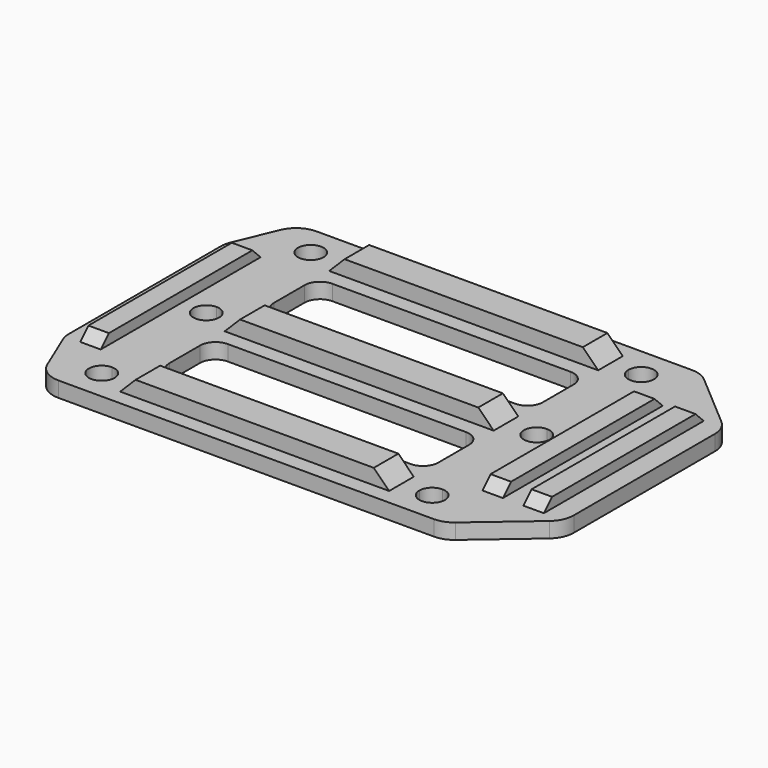
from build123d import *

# Parameters (mm, degrees)
F0_W       = 52.5
F0_H       = 3
F1_DEPTH   = 6
F0_H_2     = 6
F2_DEPTH   = 3
F4_SIZE    = 2.99999
F5_SIZE2   = 6
F5_SIZE    = 12
F5_2_SIZE2 = 6
F5_2_SIZE  = 12
F6_W       = 4
F6_H       = 39
F7_DEPTH   = 2
F8_SIZE    = 1.99999
F10_DEPTH  = 3
F13_DEPTH  = 3
F12_W      = 4
F12_H      = 39
F15_DEPTH  = 2
F16_SIZE   = 1.99999
F17_SIZE   = 1.99999
F18_DEPTH  = 25
F19_R      = 5


# Not quite as in the source:
# - a fillet or chamfer is up to 0.001 mm smaller than in the source, because OpenCascade refuses the exact size


with BuildPart() as f1:
    # F0 (on Top) → F1 (new body)
    with BuildSketch(Plane.XY):
        with Locations((0, 27)):
            Rectangle(F0_W, F0_H)
        with Locations((0, 24)):
            Rectangle(F0_W, F0_H)
    extrude(amount=F1_DEPTH)


with BuildPart() as f1b:
    # F0 (on Top) → F1, piece 2 (new body)
    with BuildSketch(Plane.XY):
        Rectangle(F0_W, F0_H_2)
    extrude(amount=F1_DEPTH)


with BuildPart() as f1c:
    # F0 (on Top) → F1, piece 3 (new body)
    with BuildSketch(Plane.XY):
        with Locations((0, -24)):
            Rectangle(F0_W, F0_H)
        with Locations((0, -27)):
            Rectangle(F0_W, F0_H)
    extrude(amount=F1_DEPTH)


with BuildPart() as f2:
    # F0 (on Top) → F2 (new body)
    with BuildSketch(Plane.XY):
        Polygon((-38.25, 28.5), (-38.25, -28.5), (-38.25, -31.5), (-35.25, -31.5), (35.25, -31.5), (38.25, -31.5), (38.25, -28.5), (38.25, 28.5), (38.25, 31.5), (35.25, 31.5), (-35.25, 31.5), (-38.25, 31.5), align=None)
        with BuildLine():
            Line((-26.25, -25.5), (-29.75, -25.5))
            ThreePointArc((-29.75, -25.5), (-34.017766953, -27.267766953), (-32.25, -23))
            Line((-32.25, -23), (-32.25, -2.5))
            ThreePointArc((-32.25, -2.5), (-34.75, 0), (-32.25, 2.5))
            Line((-32.25, 2.5), (-32.25, 23))
            ThreePointArc((-32.25, 23), (-34.017766953, 27.267766953), (-29.75, 25.5))
            Line((-29.75, 25.5), (-26.25, 25.5))
            Line((-26.25, 25.5), (-26.25, 28.5))
            Line((-26.25, 28.5), (26.25, 28.5))
            Line((26.25, 28.5), (26.25, 25.5))
            Line((26.25, 25.5), (29.75, 25.5))
            ThreePointArc((29.75, 25.5), (32.25, 28), (34.75, 25.5))
            ThreePointArc((34.75, 25.5), (34.017766953, 23.732233047), (32.25, 23))
            Line((32.25, 23), (32.25, 2.5))
            ThreePointArc((32.25, 2.5), (34.017766953, 1.767766953), (34.75, 0))
            ThreePointArc((34.75, 0), (34.017766953, -1.767766953), (32.25, -2.5))
            Line((32.25, -2.5), (32.25, -23))
            ThreePointArc((32.25, -23), (34.017766953, -23.732233047), (34.75, -25.5))
            ThreePointArc((34.75, -25.5), (32.25, -28), (29.75, -25.5))
            Line((29.75, -25.5), (26.25, -25.5))
            Line((26.25, -25.5), (26.25, -28.5))
            Line((26.25, -28.5), (-26.25, -28.5))
            Line((-26.25, -28.5), (-26.25, -25.5))
        make_face(mode=Mode.SUBTRACT)
        with BuildLine():
            ThreePointArc((-32.25, -23), (-30.482233047, -23.732233047), (-29.75, -25.5))
            Line((-29.75, -25.5), (-26.25, -25.5))
            Line((-26.25, -25.5), (-26.25, -22.5))
            Line((-26.25, -22.5), (26.25, -22.5))
            Line((26.25, -22.5), (26.25, -25.5))
            Line((26.25, -25.5), (29.75, -25.5))
            ThreePointArc((29.75, -25.5), (30.482233047, -23.732233047), (32.25, -23))
            Line((32.25, -23), (32.25, -2.5))
            ThreePointArc((32.25, -2.5), (29.75, 0), (32.25, 2.5))
            Line((32.25, 2.5), (32.25, 23))
            ThreePointArc((32.25, 23), (30.482233047, 23.732233047), (29.75, 25.5))
            Line((29.75, 25.5), (26.25, 25.5))
            Line((26.25, 25.5), (26.25, 22.5))
            Line((26.25, 22.5), (-26.25, 22.5))
            Line((-26.25, 22.5), (-26.25, 25.5))
            Line((-26.25, 25.5), (-29.75, 25.5))
            ThreePointArc((-29.75, 25.5), (-30.482233047, 23.732233047), (-32.25, 23))
            Line((-32.25, 23), (-32.25, 2.5))
            ThreePointArc((-32.25, 2.5), (-30.482233047, 1.767766953), (-29.75, 0))
            ThreePointArc((-29.75, 0), (-30.482233047, -1.767766953), (-32.25, -2.5))
            Line((-32.25, -2.5), (-32.25, -23))
        make_face()
        with BuildLine():
            ThreePointArc((-23.25, -19.5), (-25.3713203436, -18.6213203436), (-26.25, -16.5))
            Line((-26.25, -16.5), (-26.25, -9))
            ThreePointArc((-26.25, -9), (-25.3713203436, -6.8786796564), (-23.25, -6))
            Line((-23.25, -6), (23.25, -6))
            ThreePointArc((23.25, -6), (25.3713203436, -6.8786796564), (26.25, -9))
            Line((26.25, -9), (26.25, -16.5))
            ThreePointArc((26.25, -16.5), (25.3713203436, -18.6213203436), (23.25, -19.5))
            Line((23.25, -19.5), (-23.25, -19.5))
        make_face(mode=Mode.SUBTRACT)
        Rectangle(F0_W, F0_H_2, mode=Mode.SUBTRACT)
        with BuildLine():
            Line((-23.25, 19.5), (23.25, 19.5))
            ThreePointArc((23.25, 19.5), (25.3713203436, 18.6213203436), (26.25, 16.5))
            Line((26.25, 16.5), (26.25, 9))
            ThreePointArc((26.25, 9), (25.3713203436, 6.8786796564), (23.25, 6))
            Line((23.25, 6), (-23.25, 6))
            ThreePointArc((-23.25, 6), (-25.3713203436, 6.8786796564), (-26.25, 9))
            Line((-26.25, 9), (-26.25, 16.5))
            ThreePointArc((-26.25, 16.5), (-25.3713203436, 18.6213203436), (-23.25, 19.5))
        make_face(mode=Mode.SUBTRACT)
        Polygon((-38.25, -31.5), (-38.25, -28.5), (-38.25, 28.5), (-38.25, 31.5), (-41.25, 31.5), (-44.25, 31.5), (-44.25, 28.5), (-44.25, -28.5), (-44.25, -31.5), (-41.25, -31.5), align=None)
        Polygon((38.25, -28.5), (38.25, -31.5), (41.25, -31.5), (44.25, -31.5), (44.25, -28.5), (44.25, 28.5), (44.25, 31.5), (41.25, 31.5), (38.25, 31.5), (38.25, 28.5), align=None)
    extrude(amount=F2_DEPTH)


with BuildPart() as f1c_1:
    add(f1c.part)

    # F3: union F1, F1b, F2
    add(f1.part)
    add(f1b.part)
    add(f2.part)

    # F4 (size 3 in the source; OpenCascade refuses exactly that, so slightly less here)
    f4_edges = [f1c_1.edges().sort_by_distance(p)[0] for p in [
        (26.25, 25.5, 6),
        (26.25, 0, 6),
        (26.25, -25.5, 6),
        (-26.25, 25.5, 6),
        (-26.25, 0, 6),
        (-26.25, -25.5, 6),
    ]]
    chamfer(f4_edges, length=F4_SIZE)

    # F5
    f5_edges = [f1c_1.edges().sort_by_distance(p)[0] for p in [
        (44.25, -31.5, 1.5),
        (44.25, 31.5, 1.5),
    ]]
    f5_side = f1c_1.faces().sort_by_distance((44.25, 0, 1.5))[0]
    chamfer(f5_edges, length=F5_SIZE, length2=F5_SIZE2, reference=f5_side)

    # F5#2
    f5_2_edges = [f1c_1.edges().sort_by_distance(p)[0] for p in [
        (-44.25, -31.5, 1.5),
        (-44.25, 31.5, 1.5),
    ]]
    f5_2_side = f1c_1.faces().sort_by_distance((-44.25, 0, 1.5))[0]
    chamfer(f5_2_edges, length=F5_2_SIZE, length2=F5_2_SIZE2, reference=f5_2_side)

    # F6 (on face) → F7 (join)
    with BuildSketch(Plane.XY.offset(3)):
        with Locations((-39.25, 0)):
            Rectangle(F6_W, F6_H)
        with Locations((39.25, 0)):
            Rectangle(F6_W, F6_H)
    extrude(amount=F7_DEPTH)

    # F8 (size 2 in the source; OpenCascade refuses exactly that, so slightly less here)
    f8_edges = [f1c_1.edges().sort_by_distance(p)[0] for p in [
        (-39.25, -19.5, 5),
        (-39.25, 19.5, 5),
        (39.25, 19.5, 5),
        (39.25, -19.5, 5),
    ]]
    chamfer(f8_edges, length=F8_SIZE)


with BuildPart() as f10:
    # F9 (on face) → F10 (new body)
    with BuildSketch(Plane(origin=(0, 0, 0), x_dir=(1, 0, 0), z_dir=(0, 0, -1))):
        Polygon((53.25, 31.5), (38.25, 31.5), (44.25, 19.5), (44.25, -19.5), (38.25, -31.5), (53.25, -31.5), align=None)
    extrude(amount=-F10_DEPTH)


with BuildPart() as f1c_2:
    add(f1c_1.part)

    # F11: union F10
    add(f10.part)


with BuildPart() as f13:
    # F12 (on face) → F13 (new body)
    with BuildSketch(Plane.XY.offset(3)):
        Polygon((-38.25, -31.5), (-44.25, -19.5), (-39.25, -31.5), align=None)
    extrude(amount=-F13_DEPTH)


with BuildPart() as f13b:
    # F12 (on face) → F13, piece 2 (new body)
    with BuildSketch(Plane.XY.offset(3)):
        Polygon((-38.25, 31.5), (-39.25, 31.5), (-44.25, 19.5), align=None)
    extrude(amount=-F13_DEPTH)


with BuildPart() as f1c_3:
    add(f1c_2.part)

    # F14: union F13b, F13
    add(f13b.part)
    add(f13.part)

    # F12 (on face) → F15 (join)
    with BuildSketch(Plane.XY.offset(3)):
        with Locations((47.25, 0)):
            Rectangle(F12_W, F12_H)
    extrude(amount=F15_DEPTH)

    # F16 (size 2 in the source; OpenCascade refuses exactly that, so slightly less here)
    f16_edges = [f1c_3.edges().sort_by_distance(p)[0] for p in [
        (47.25, -19.5, 5),
    ]]
    chamfer(f16_edges, length=F16_SIZE)

    # F17 (size 2 in the source; OpenCascade refuses exactly that, so slightly less here)
    f17_edges = [f1c_3.edges().sort_by_distance(p)[0] for p in [
        (47.25, 19.5, 5),
    ]]
    chamfer(f17_edges, length=F17_SIZE)

    # F12 (on face) → F18 (cut)
    with BuildSketch(Plane.XY.offset(3)):
        Polygon((53.25, 31.5), (39.25, 31.5), (53.25, 19.5), align=None)
        Polygon((53.25, -19.5), (39.25, -31.5), (53.25, -31.5), align=None)
    extrude(amount=-F18_DEPTH, mode=Mode.SUBTRACT)

    # F19
    f19_edges = [f1c_3.edges().sort_by_distance(p)[0] for p in [
        (39.25, -31.5, 1.5),
        (53.25, -19.5, 1.5),
        (-39.25, -31.5, 1.5),
        (-44.25, -19.5, 1.5),
        (-44.25, 19.5, 1.5),
        (-39.25, 31.5, 1.5),
        (39.25, 31.5, 1.5),
        (53.25, 19.5, 1.5),
    ]]
    fillet(f19_edges, radius=F19_R)


solid = f1c_3.part
